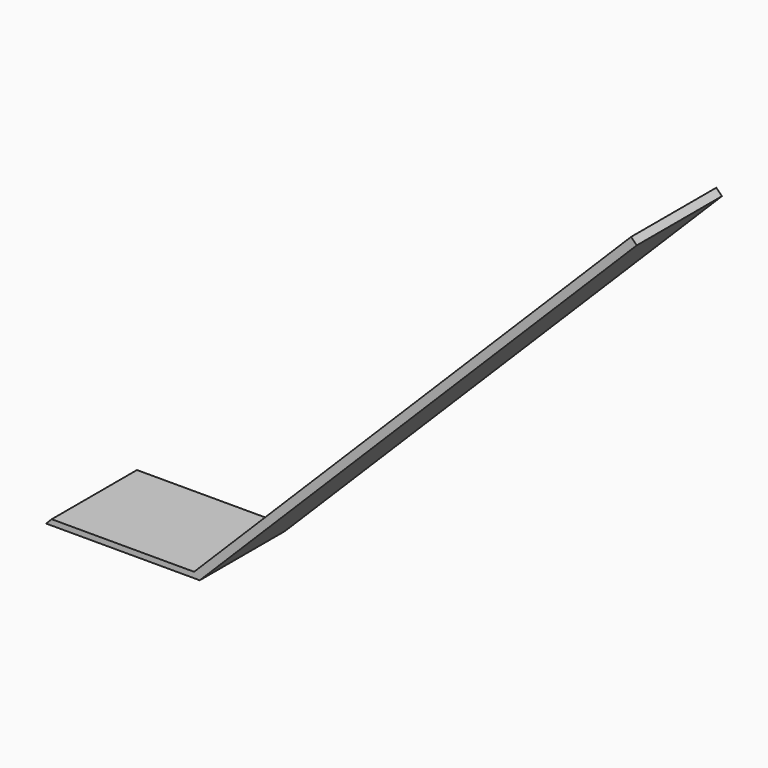
from build123d import *

# Parameters (mm, degrees)
F1_DEPTH    = 254
F2_T1_DEPTH = 332.3831903594
F3_R        = 5.08


# Not quite as in the source:
# - a fillet or chamfer that OpenCascade refuses, or shapes differently, is made with other operations: its cross-section is extruded or revolved along the edge and cut away or added


with BuildPart() as f1:
    # F0 (on Front) → F1 (new body)
    with BuildSketch(Plane.XZ):
        Polygon((1041.7304627271, 1041.6889569475), (0, 0), (-354.6740262396, 0), (-354.6520841774, -13.4706525353), (13.4701158226, -13.4706525353), (1055.2005785497, 1028.2183044122), align=None)
    extrude(amount=F1_DEPTH)

    # F2: chamfer of 15.24 on 1 edges, made by hand

    # F2_s2 → F2_t1 (cut)
    with BuildSketch(Plane.XZ.offset(-39.1915951797)):
        Polygon((-339.4340262396, 0), (-354.6492021575, -15.2399797823), (-354.6740262396, 0), align=None)
    extrude(amount=F2_T1_DEPTH, mode=Mode.SUBTRACT)

    # F3
    f3_edges = [f1.edges().sort_by_distance(p)[0] for p in [
        (0, -127, 0),
    ]]
    fillet(f3_edges, radius=F3_R)


solid = f1.part
